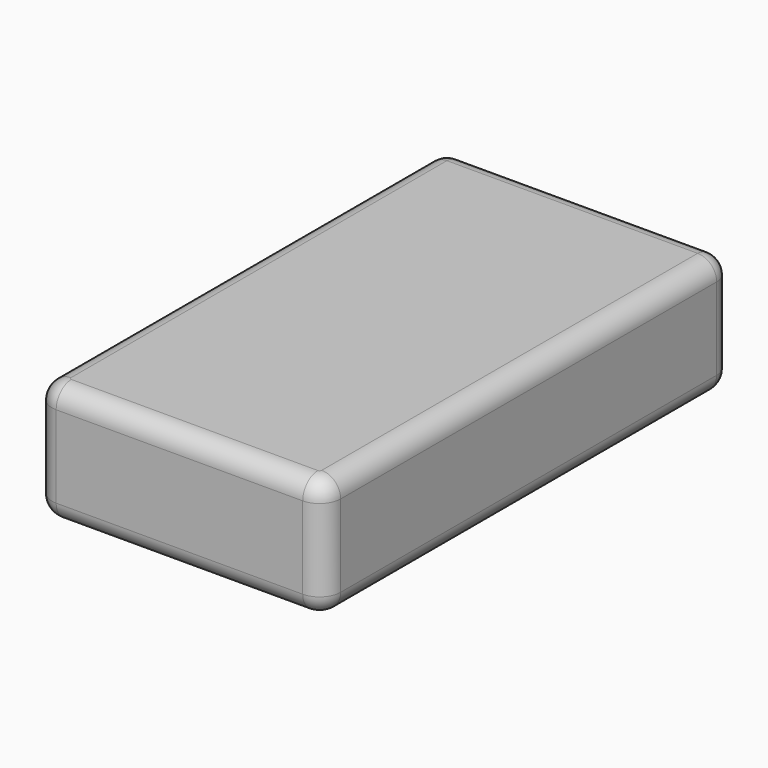
from build123d import *

# Parameters (mm, degrees)
F1_DEPTH    = 2.85
F2_DEPTH    = 1.95
F3_DEPTH    = 2.85
F4_DEPTH    = 1.95
F5_R        = 1
F7_DEPTH    = 25
F8_T1_DEPTH = 11.9
F9_R        = 0.89999


# Not quite as in the source:
# - a fillet or chamfer that OpenCascade refuses, or shapes differently, is made with other operations: its cross-section is extruded or revolved along the edge and cut away or added
# - a fillet or chamfer is up to 0.001 mm smaller than in the source, because OpenCascade refuses the exact size


with BuildPart() as f1:
    # F0 (on Top) → F1 (new body)
    with BuildSketch(Plane.XY):
        Polygon((-5.95, 11.2), (-5.95, -11.2), (5.95, -11.2), (5.95, 11.2), (5.95, 12.1), (-5.95, 12.1), align=None)
        Polygon((5.95, -11.2), (-5.95, -11.2), (-5.95, 11.2), (-5.95, 12.1), (-6.85, 12.1), (-6.85, -12.1), (6.85, -12.1), (6.85, 12.1), (5.95, 12.1), (5.95, 11.2), align=None)
    extrude(amount=F1_DEPTH)

    # F0 (on Top) → F2 (cut)
    with BuildSketch(Plane.XY):
        Polygon((-5.95, 11.2), (-5.95, -11.2), (5.95, -11.2), (5.95, 11.2), (5.95, 12.1), (-5.95, 12.1), align=None)
    extrude(amount=F2_DEPTH, mode=Mode.SUBTRACT)

    # F0 (on Top) → F3 (join)
    with BuildSketch(Plane.XY):
        Polygon((-5.95, 11.2), (-5.95, -11.2), (5.95, -11.2), (5.95, 11.2), (5.95, 12.1), (-5.95, 12.1), align=None)
        Polygon((5.95, -11.2), (-5.95, -11.2), (-5.95, 11.2), (-5.95, 12.1), (-6.85, 12.1), (-6.85, -12.1), (6.85, -12.1), (6.85, 12.1), (5.95, 12.1), (5.95, 11.2), align=None)
    extrude(amount=-F3_DEPTH)

    # F0 (on Top) → F4 (cut)
    with BuildSketch(Plane.XY):
        Polygon((-5.95, 11.2), (-5.95, -11.2), (5.95, -11.2), (5.95, 11.2), (5.95, 12.1), (-5.95, 12.1), align=None)
    extrude(amount=-F4_DEPTH, mode=Mode.SUBTRACT)

    # F5
    f5_edges = [f1.edges().sort_by_distance(p)[0] for p in [
        (5.95, -11.2, 0),
        (-5.95, -11.2, 0),
        (-6.85, -12.1, 0),
        (6.85, -12.1, 0),
    ]]
    fillet(f5_edges, radius=F5_R)

    # F6 (on Top) → F7 (cut)
    with BuildSketch(Plane.XY):
        Polygon((-5.95, 1), (-5.95, -4), (5.95, -4), (5.95, 1), (0, 1), align=None)
    extrude(amount=-F7_DEPTH, mode=Mode.SUBTRACT)

    # F8: chamfer of 2 on 2 edges, made by hand

    # F8_s2 → F8_t1 (cut)
    with BuildSketch(Plane.YZ.offset(-5.95)):
        Polygon((-6, -2.85), (-4, -0.85), (-4, -2.85), align=None)
        Polygon((3, -2.85), (1, -0.85), (1, -2.85), align=None)
    extrude(amount=F8_T1_DEPTH, mode=Mode.SUBTRACT)

    # F9 (radius 0.9 in the source; OpenCascade refuses exactly that, so slightly less here)
    f9_edges = [f1.edges().sort_by_distance(p)[0] for p in [
        (6.85, 12.1, 0),
        (-6.85, 12.1, 0),
        (0, 12.1, -2.85),
        (0, 12.1, 2.85),
        (6.85, 0.5, -2.85),
        (0, -12.1, 2.85),
        (-6.85, 0.5, 2.85),
        (-6.85, 0.5, -2.85),
        (-6.557107, -11.807107, -2.85),
        (0, -12.1, -2.85),
        (6.557107, -11.807107, -2.85),
        (6.85, 0.5, 2.85),
        (6.557107, -11.807107, 2.85),
        (-6.557107, -11.807107, 2.85),
    ]]
    fillet(f9_edges, radius=F9_R)


solid = f1.part
